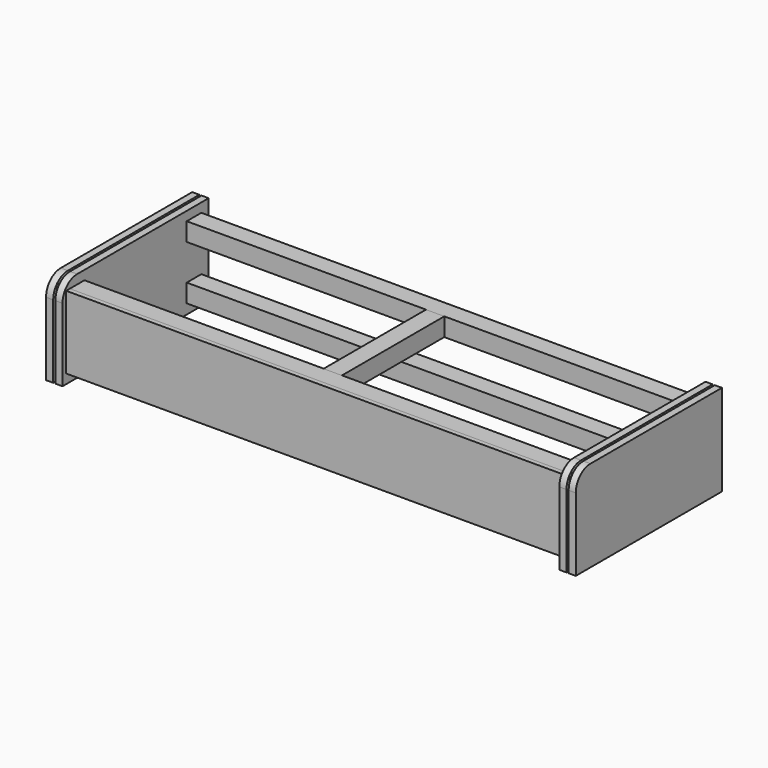
from build123d import *

# Parameters (mm, degrees)
F1_DEPTH  = 18
F2_W      = 2.4
F2_H      = 92.5
F3_DEPTH  = 7.5
F2_H_2    = 7.5
F4_DEPTH  = 200
F5_R      = 20
F0_W      = 10
F0_H      = 10
F0_H_2    = 10.8381873609
F6_DEPTH  = 7.8
F12_DEPTH = 564.4
F13_W     = 564.4
F13_H     = 79.7317819297
F14_DEPTH = 5
F15_W     = 20
F15_H     = 140.1707154512
F16_DEPTH = 20


# Not quite as in the source:
# - a feature names something its author has since deleted; it is built from what else it names


with BuildPart() as f1:
    # F0 (on Right) → F1 (new body)
    with BuildSketch(Plane.YZ):
        Polygon((16.6586227824, -50), (100, -50), (100, -5.0102403117), (100, 5.0102403117), (100, 50), (14.8988555628, 50), (-16.6586227824, 50), (-100, 50), (-100, 5.0102403117), (-100, -5.0102403117), (-100, -50), (-14.8988555628, -50), align=None)
        Polygon((70, -39.1618126391), (70, -30), (-70, -30), (-70, -40), (-90, -40), (-90, -36.8431898768), (-90, -20), (-80, -20), (-80, 14.1863731473), (-80, 20), (-90, 20), (-90, 40), (-70, 40), (-70, 30), (70, 30), (70, 40), (90, 40), (90, 20), (80, 20), (80, -19.1618126391), (90, -19.1618126391), (90, -39.1618126391), align=None, mode=Mode.SUBTRACT)
        Polygon((-70, -30), (70, -30), (70, -19.1618126391), (80, -19.1618126391), (80, 20), (70, 20), (70, 30), (-70, 30), (-70, 20), (-80, 20), (-80, 14.1863731473), (-80, -20), (-70, -20), align=None)
    extrude(amount=-F1_DEPTH)

    # F2 (on face) → F3 (cut)
    with BuildSketch(Plane.XZ.offset(100)):
        with Locations((-9, -3.75)):
            Rectangle(F2_W, F2_H)
    extrude(amount=-F3_DEPTH, mode=Mode.SUBTRACT)

    # F2 (on face) → F4 (cut, through all)
    with BuildSketch(Plane.XZ.offset(100)):
        with Locations((-9, 46.25)):
            Rectangle(F2_W, F2_H_2)
    extrude(amount=-F4_DEPTH, mode=Mode.SUBTRACT)

    # F5
    f5_edges = [f1.edges().sort_by_distance(p)[0] for p in [
        (-3.9, -100, 50),
        (-14.1, -100, 50),
    ]]
    fillet(f5_edges, radius=F5_R)

    # F0 (on Right) → F6 (join, through all)
    with BuildSketch(Plane.YZ):
        Polygon((80, 30), (80, 20), (90, 20), (90, 40), (70, 40), (70, 30), align=None)
        with Locations((75, 25)):
            Rectangle(F0_W, F0_H)
        Polygon((-80, 30), (-70, 30), (-70, 40), (-90, 40), (-90, 20), (-80, 20), align=None)
        with Locations((-75, 25)):
            Rectangle(F0_W, F0_H)
        with Locations((-75, -25)):
            Rectangle(F0_W, F0_H)
        Polygon((-70, -40), (-70, -30), (-80, -30), (-80, -20), (-90, -20), (-90, -36.8431898768), (-90, -40), align=None)
        Polygon((80, -19.1618126391), (80, -30), (70, -30), (70, -39.1618126391), (90, -39.1618126391), (90, -19.1618126391), align=None)
        with Locations((75, -24.5809063196)):
            Rectangle(F0_W, F0_H_2)
    extrude(amount=-F6_DEPTH)


with BuildPart() as f7_1:
    # F7: copy of F1
    add(f1.part)


with BuildPart() as f9_1:
    # F9: copy of F1
    add(f1.part.moved(Location((-580, 0, 0))))


with BuildPart() as f10_1:
    # F10: instance of F9_1
    add(f9_1.part.mirror(Plane(origin=(-580, 0.4117970533, -0.1962701674), x_dir=(0, 1, 0), z_dir=(1, 0, 0))))


with BuildPart() as f12:
    # F12 (new, through all): a face of the model
    f12_faces = [f10_1.part.faces().sort_by_distance(p)[0] for p in [
        (-572.2, 80, 30),
    ]]
    extrude(f12_faces, amount=F12_DEPTH)


with BuildPart() as f12b:
    # F12#2 (new, through all): a face of the model
    f12_2_faces = [f10_1.part.faces().sort_by_distance(p)[0] for p in [
        (-572.2, -80, 30),
    ]]
    extrude(f12_2_faces, amount=F12_DEPTH)


with BuildPart() as f12c:
    # F12#3 (new, through all): a face of the model
    f12_3_faces = [f10_1.part.faces().sort_by_distance(p)[0] for p in [
        (-572.2, -80, -30),
    ]]
    extrude(f12_3_faces, amount=F12_DEPTH)


with BuildPart() as f12d:
    # F12#4 (new, through all): a face of the model
    f12_4_faces = [f10_1.part.faces().sort_by_distance(p)[0] for p in [
        (-572.2, 80, -29.1618126391),
    ]]
    extrude(f12_4_faces, amount=F12_DEPTH)


with BuildPart() as f14:
    # F13 (on face) → F14 (new body)
    with BuildSketch(Plane.XZ.offset(90)):
        with Locations((-290, 0.1341090351)):
            Rectangle(F13_W, F13_H)
    extrude(amount=F14_DEPTH)


with BuildPart() as f16:
    # F15 (on face) → F16 (new body)
    with BuildSketch(Plane.XY.offset(40)):
        with Locations((-290, -0.0853577256)):
            Rectangle(F15_W, F15_H)
    extrude(amount=-F16_DEPTH)


solid = Compound([f1.part, f10_1.part, f12.part, f12b.part, f12c.part, f12d.part, f14.part, f16.part])
